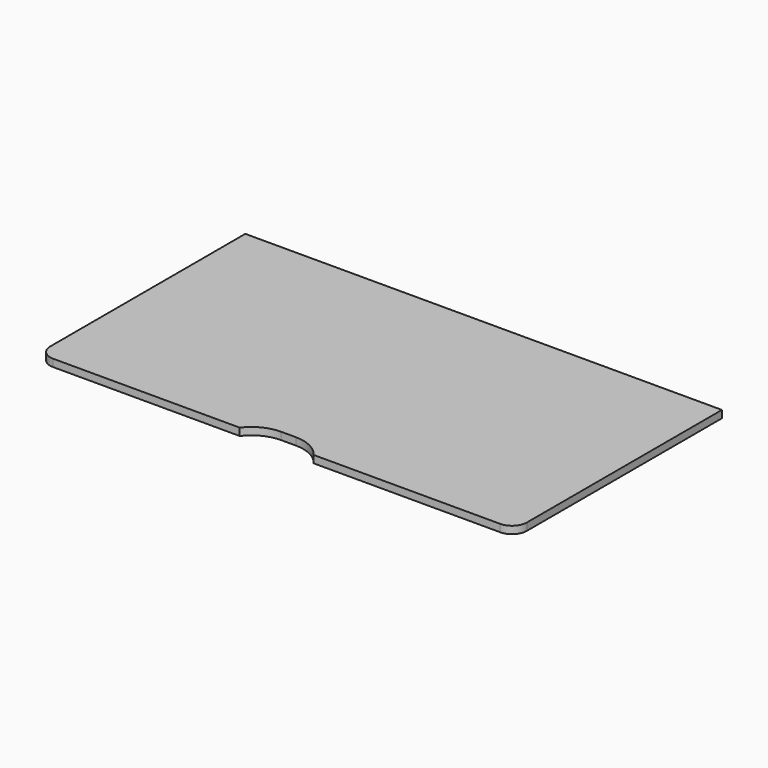
from build123d import *

# Parameters (mm, degrees)
F0_W        = 64.5
F0_H        = 35
F1_DEPTH    = 1
F2_R        = 2
F3_W        = 10
F3_H        = 1
F4_DEPTH    = 2
F5_T1_DEPTH = 1


# Not quite as in the source:
# - a fillet or chamfer that OpenCascade refuses, or shapes differently, is made with other operations: its cross-section is extruded or revolved along the edge and cut away or added


with BuildPart() as f1:
    # F0 (on Top) → F1 (new body)
    with BuildSketch(Plane.XY):
        with Locations((0, -0.7672849298)):
            Rectangle(F0_W, F0_H)
    extrude(amount=F1_DEPTH)

    # F2
    f2_edges = [f1.edges().sort_by_distance(p)[0] for p in [
        (-32.25, -18.267285, 0.5),
        (32.25, -18.267285, 0.5),
    ]]
    fillet(f2_edges, radius=F2_R)

    # F3 (on face) → F4 (cut)
    with BuildSketch(Plane.XZ.offset(18.2672849298)):
        with Locations((0, 0.5)):
            Rectangle(F3_W, F3_H)
    extrude(amount=-F4_DEPTH, mode=Mode.SUBTRACT)

    # F5: fillet of radius 5 on 2 edges, made by hand

    # F5_s2 → F5_t1 (join)
    with BuildSketch(Plane.XY):
        with BuildLine():
            ThreePointArc((5, -18.2672849298), (3.2360679775, -16.7951489748), (1, -16.2672849298))
            Line((1, -16.2672849298), (5, -16.2672849298))
            Line((5, -16.2672849298), (5, -18.2672849298))
        make_face()
        with BuildLine():
            ThreePointArc((-1, -16.2672849298), (-3.2360679775, -16.7951489748), (-5, -18.2672849298))
            Line((-5, -18.2672849298), (-5, -16.2672849298))
            Line((-5, -16.2672849298), (-1, -16.2672849298))
        make_face()
    extrude(amount=F5_T1_DEPTH)


solid = f1.part
